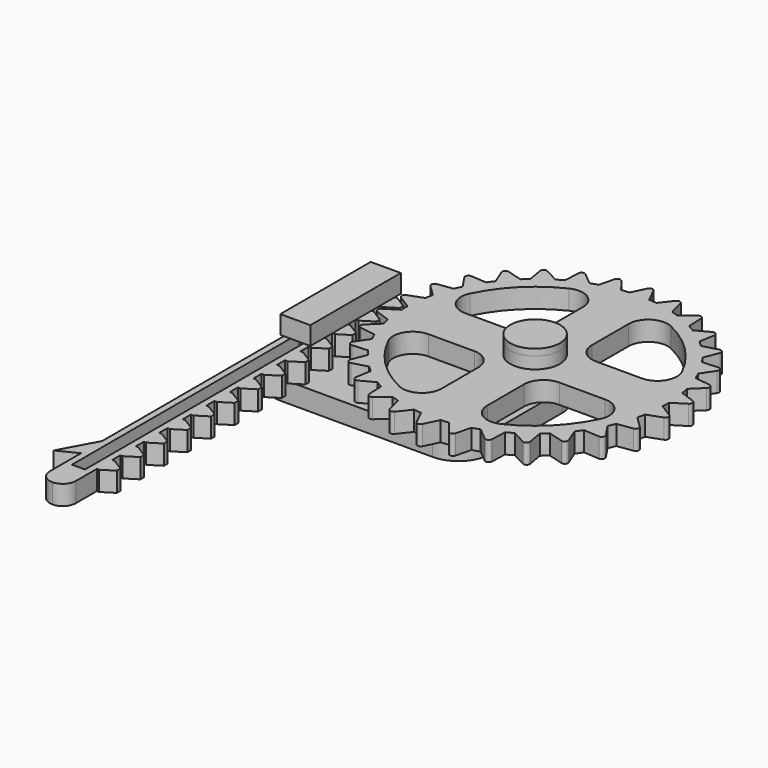
from build123d import *

# Parameters (mm, degrees)
F1_DEPTH        = 3
F2_DEPTH        = 3
F2_COPIES_COUNT = 30
F3_R            = 0.5
F5_DEPTH        = 3
F6_W            = 2
F6_H            = 57.4811261014
F7_DEPTH        = 3.001
F8_T1_DEPTH     = 12.7063351407
F8_T3_DEPTH     = 13
F9_R            = 18
F10_DEPTH       = 3.001
F11_W           = 15
F11_H           = 7
F11_W_2         = 7
F11_H_2         = 15
F12_DEPTH       = 3
F13_R           = 2.5
F14_DEPTH       = 3.001
F15_R           = 3
F16_W           = 33.1953612559
F16_H           = 23.5
F17_DEPTH       = 3
F18_W           = 1.3
F18_H           = 14
F19_DEPTH       = 5
F20_R           = 5
F21_R           = 2.15
F22_DEPTH       = 5
F23_R           = 3.8
F23_R_2         = 2.3
F24_DEPTH       = 1.8
F25_R           = 3.8
F26_DEPTH       = 1
F27_W           = 4.6
F27_H           = 17.3
F27_W_2         = 1.6
F27_H_2         = 14.3
F28_DEPTH       = 1.8
F29_W           = 4.6
F29_H           = 17.3
F30_DEPTH       = 1
F32_DEPTH       = 3
F34_DEPTH       = 3
F35_W           = 1
F35_H           = 1
F36_DEPTH       = 1


# Not quite as in the source:
# - a fillet or chamfer that OpenCascade refuses, or shapes differently, is made with other operations: its cross-section is extruded or revolved along the edge and cut away or added
# - a pattern or mirror of a feature is missing from the dataset's text; its kind, count and spacing are read off the source's solid


with BuildPart() as f1:
    # F0 (on Top) → F1 (new body)
    with BuildSketch(Plane.XY):
        with BuildLine():
            ThreePointArc((-1.5, 19.9436706752), (-13.6014705087, -14.6628782986), (20, 0))
            ThreePointArc((20, 0), (14.6628782986, 13.6014705087), (1.5, 19.9436706752))
            ThreePointArc((1.5, 19.9436706752), (0, 20), (-1.5, 19.9436706752))
        make_face()
    extrude(amount=F1_DEPTH)

    # F0 (on Top) → F2 (join)
    with BuildSketch(Plane.XY):
        with BuildLine():
            ThreePointArc((-1.5, 19.9436706752), (0, 20), (1.5, 19.9436706752))
            Line((1.5, 19.9436706752), (0, 23))
            Line((0, 23), (-1.5, 19.9436706752))
        make_face()
    f2 = extrude(amount=F2_DEPTH)

    # F2_copies: F2 ×30 about axis
    f2_copies_axis = Axis((0, 0, 0), (0, 0, 1))
    for i in range(1, F2_COPIES_COUNT):
        add(f2.rotate(f2_copies_axis, i * 360 / F2_COPIES_COUNT))

    # F3
    f3_edges = [f1.edges().sort_by_distance(p)[0] for p in [
        (0, 23, 1.5),
        (22.874004, -2.404155, 1.5),
        (22.874004, 2.404155, 1.5),
        (21.8743, 7.107391, 1.5),
        (19.918584, 11.5, 1.5),
        (17.092331, 15.390004, 1.5),
        (13.519061, 18.607391, 1.5),
        (9.354943, 21.011546, 1.5),
        (-4.781969, 22.497395, 1.5),
        (-9.354943, 21.011546, 1.5),
        (-13.519061, 18.607391, 1.5),
        (-17.092331, 15.390004, 1.5),
        (-19.918584, 11.5, 1.5),
        (-21.8743, 7.107391, 1.5),
        (-22.874004, 2.404155, 1.5),
        (-22.874004, -2.404155, 1.5),
        (-21.8743, -7.107391, 1.5),
        (-19.918584, -11.5, 1.5),
        (-17.092331, -15.390004, 1.5),
        (-13.519061, -18.607391, 1.5),
        (-9.354943, -21.011546, 1.5),
        (-4.781969, -22.497395, 1.5),
        (0, -23, 1.5),
        (4.781969, -22.497395, 1.5),
        (9.354943, -21.011546, 1.5),
        (13.519061, -18.607391, 1.5),
        (17.092331, -15.390004, 1.5),
        (19.918584, -11.5, 1.5),
        (21.8743, -7.107391, 1.5),
        (4.781969, 22.497395, 1.5),
    ]]
    fillet(f3_edges, radius=F3_R)

    # F9 (on face) → F10 (cut, through all)
    with BuildSketch(Plane.XY.offset(3)):
        Circle(F9_R)
    extrude(amount=-F10_DEPTH, mode=Mode.SUBTRACT)

    # F11 (on Top) → F12 (join)
    with BuildSketch(Plane.XY):
        with Locations((-11, 0)):
            Rectangle(F11_W, F11_H)
        with Locations((0, 11)):
            Rectangle(F11_W_2, F11_H_2)
        Rectangle(F11_W_2, F11_H)
        with Locations((0, -11)):
            Rectangle(F11_W_2, F11_H_2)
        with Locations((11, 0)):
            Rectangle(F11_W, F11_H)
    extrude(amount=F12_DEPTH)

    # F13 (on face) → F14 (cut, through all)
    with BuildSketch(Plane.XY.offset(3)):
        Circle(F13_R)
    extrude(amount=-F14_DEPTH, mode=Mode.SUBTRACT)

    # F15
    f15_edges = [f1.edges().sort_by_distance(p)[0] for p in [
        (3.5, 17.656444, 1.5),
        (3.5, -3.5, 1.5),
        (-3.5, -3.5, 1.5),
        (17.656444, -3.5, 1.5),
        (3.5, -17.656444, 1.5),
        (-17.656444, -3.5, 1.5),
        (-3.5, -17.656444, 1.5),
        (-3.5, 3.5, 1.5),
        (3.5, 3.5, 1.5),
        (-17.656444, 3.5, 1.5),
        (-3.5, 17.656444, 1.5),
        (17.656444, 3.5, 1.5),
    ]]
    fillet(f15_edges, radius=F15_R)


with BuildPart() as f5:
    # F4 (on Top) → F5 (new body)
    with BuildSketch(Plane.XY):
        Polygon((-26.6953612559, 3), (-26.6953612559, -61.4811261014), (-22.6953612559, -61.4811261014), (-22.6953612559, -55.4810394768), (-22.6953612559, -52.518787274), (-22.6953612559, -50.9810466955), (-22.6953612559, -48.0187944927), (-22.6953612559, -46.4810539142), (-22.6953612559, -43.5188017114), (-22.6953612559, -41.9810611329), (-22.6953612559, -39.0188089301), (-22.6953612559, -37.4810683516), (-22.6953612559, -34.5188161489), (-22.6953612559, -32.9810755704), (-22.6953612559, -30.0188233676), (-22.6953612559, -28.4810827891), (-22.6953612559, -25.5188305863), (-22.6953612559, -23.9810900078), (-22.6953612559, -21.018837805), (-22.6953612559, -19.4810972265), (-22.6953612559, -16.5188450237), (-22.6953612559, -14.9811044452), (-22.6953612559, -12.0188522425), (-22.6953612559, -10.4811116639), (-22.6953612559, -7.5188594612), (-22.6953612559, -5.9811188827), (-22.6953612559, -3.0188666799), (-22.6953612559, -1.4811261014), (-22.6953612559, 1.4811261014), (-22.6953612559, 3), align=None)
        with BuildLine():
            Line((-22.6953612559, -52.518787274), (-22.6953612559, -55.4810394768))
            Line((-22.6953612559, -55.4810394768), (-22.3474906883, -55.4810394768))
            Line((-22.3474906883, -55.4810394768), (-20.5437649967, -54.3477605362))
            ThreePointArc((-20.5437649967, -54.3477605362), (-20.5467235884, -53.9999133754), (-20.5437649967, -53.6520662145))
            Line((-20.5437649967, -53.6520662145), (-22.3474906883, -52.518787274))
            Line((-22.3474906883, -52.518787274), (-22.6953612559, -52.518787274))
        make_face()
        with BuildLine():
            Line((-22.2507670999, 1.4811261014), (-22.6953612559, 1.4811261014))
            Line((-22.6953612559, 1.4811261014), (-22.6953612559, -1.4811261014))
            Line((-22.6953612559, -1.4811261014), (-22.2507670999, -1.4811261014))
            Line((-22.2507670999, -1.4811261014), (-20.4470414083, -0.3478471608))
            ThreePointArc((-20.4470414083, -0.3478471608), (-20.45, 0), (-20.4470414083, 0.3478471608))
            Line((-20.4470414083, 0.3478471608), (-22.2507670999, 1.4811261014))
        make_face()
        with BuildLine():
            Line((-22.6953612559, -48.0187944927), (-22.6953612559, -50.9810466955))
            Line((-22.6953612559, -50.9810466955), (-22.3394303893, -50.9810466955))
            Line((-22.3394303893, -50.9810466955), (-20.5357046977, -49.8477677549))
            ThreePointArc((-20.5357046977, -49.8477677549), (-20.5386632894, -49.4999205941), (-20.5357046977, -49.1520734333))
            Line((-20.5357046977, -49.1520734333), (-22.3394303893, -48.0187944927))
            Line((-22.3394303893, -48.0187944927), (-22.6953612559, -48.0187944927))
        make_face()
        with BuildLine():
            Line((-22.2588273989, -3.0188666799), (-22.6953612559, -3.0188666799))
            Line((-22.6953612559, -3.0188666799), (-22.6953612559, -5.9811188827))
            Line((-22.6953612559, -5.9811188827), (-22.2588273989, -5.9811188827))
            Line((-22.2588273989, -5.9811188827), (-20.4551017073, -4.8478399421))
            ThreePointArc((-20.4551017073, -4.8478399421), (-20.458060299, -4.4999927813), (-20.4551017073, -4.1521456204))
            Line((-20.4551017073, -4.1521456204), (-22.2588273989, -3.0188666799))
        make_face()
        with BuildLine():
            Line((-22.6953612559, -43.5188017114), (-22.6953612559, -46.4810539142))
            Line((-22.6953612559, -46.4810539142), (-22.3313700903, -46.4810539142))
            Line((-22.3313700903, -46.4810539142), (-20.5276443986, -45.3477749736))
            ThreePointArc((-20.5276443986, -45.3477749736), (-20.5306029903, -44.9999278128), (-20.5276443986, -44.652080652))
            Line((-20.5276443986, -44.652080652), (-22.3313700903, -43.5188017114))
            Line((-22.3313700903, -43.5188017114), (-22.6953612559, -43.5188017114))
        make_face()
        with BuildLine():
            Line((-22.266887698, -7.5188594612), (-22.6953612559, -7.5188594612))
            Line((-22.6953612559, -7.5188594612), (-22.6953612559, -10.4811116639))
            Line((-22.6953612559, -10.4811116639), (-22.266887698, -10.4811116639))
            Line((-22.266887698, -10.4811116639), (-20.4631620064, -9.3478327234))
            ThreePointArc((-20.4631620064, -9.3478327234), (-20.4661205981, -8.9999855626), (-20.4631620064, -8.6521384017))
            Line((-20.4631620064, -8.6521384017), (-22.266887698, -7.5188594612))
        make_face()
        with BuildLine():
            Line((-22.6953612559, -39.0188089301), (-22.6953612559, -41.9810611329))
            Line((-22.6953612559, -41.9810611329), (-22.3233097912, -41.9810611329))
            Line((-22.3233097912, -41.9810611329), (-20.5195840996, -40.8477821924))
            ThreePointArc((-20.5195840996, -40.8477821924), (-20.5225426913, -40.4999350315), (-20.5195840996, -40.1520878707))
            Line((-20.5195840996, -40.1520878707), (-22.3233097912, -39.0188089301))
            Line((-22.3233097912, -39.0188089301), (-22.6953612559, -39.0188089301))
        make_face()
        with BuildLine():
            Line((-22.274947997, -12.0188522425), (-22.6953612559, -12.0188522425))
            Line((-22.6953612559, -12.0188522425), (-22.6953612559, -14.9811044452))
            Line((-22.6953612559, -14.9811044452), (-22.274947997, -14.9811044452))
            Line((-22.274947997, -14.9811044452), (-20.4712223054, -13.8478255047))
            ThreePointArc((-20.4712223054, -13.8478255047), (-20.4741808971, -13.4999783438), (-20.4712223054, -13.152131183))
            Line((-20.4712223054, -13.152131183), (-22.274947997, -12.0188522425))
        make_face()
        with BuildLine():
            Line((-22.6953612559, -34.5188161489), (-22.6953612559, -37.4810683516))
            Line((-22.6953612559, -37.4810683516), (-22.3152494922, -37.4810683516))
            Line((-22.3152494922, -37.4810683516), (-20.5115238006, -36.3477894111))
            ThreePointArc((-20.5115238006, -36.3477894111), (-20.5144823923, -35.9999422502), (-20.5115238006, -35.6520950894))
            Line((-20.5115238006, -35.6520950894), (-22.3152494922, -34.5188161489))
            Line((-22.3152494922, -34.5188161489), (-22.6953612559, -34.5188161489))
        make_face()
        with BuildLine():
            Line((-22.2830082961, -16.5188450237), (-22.6953612559, -16.5188450237))
            Line((-22.6953612559, -16.5188450237), (-22.6953612559, -19.4810972265))
            Line((-22.6953612559, -19.4810972265), (-22.2830082961, -19.4810972265))
            Line((-22.2830082961, -19.4810972265), (-20.4792826044, -18.347818286))
            ThreePointArc((-20.4792826044, -18.347818286), (-20.4822411961, -17.9999711251), (-20.4792826044, -17.6521239643))
            Line((-20.4792826044, -17.6521239643), (-22.2830082961, -16.5188450237))
        make_face()
        with BuildLine():
            Line((-22.6953612559, -30.0188233676), (-22.6953612559, -32.9810755704))
            Line((-22.6953612559, -32.9810755704), (-22.3071891932, -32.9810755704))
            Line((-22.3071891932, -32.9810755704), (-20.5034635015, -31.8477966298))
            ThreePointArc((-20.5034635015, -31.8477966298), (-20.5064220932, -31.499949469), (-20.5034635015, -31.1521023081))
            Line((-20.5034635015, -31.1521023081), (-22.3071891932, -30.0188233676))
            Line((-22.3071891932, -30.0188233676), (-22.6953612559, -30.0188233676))
        make_face()
        with BuildLine():
            Line((-22.2910685951, -21.018837805), (-22.6953612559, -21.018837805))
            Line((-22.6953612559, -21.018837805), (-22.6953612559, -23.9810900078))
            Line((-22.6953612559, -23.9810900078), (-22.2910685951, -23.9810900078))
            Line((-22.2910685951, -23.9810900078), (-20.4873429035, -22.8478110672))
            ThreePointArc((-20.4873429035, -22.8478110672), (-20.4903014952, -22.4999639064), (-20.4873429035, -22.1521167456))
            Line((-20.4873429035, -22.1521167456), (-22.2910685951, -21.018837805))
        make_face()
        with BuildLine():
            Line((-22.6953612559, -25.5188305863), (-22.6953612559, -28.4810827891))
            Line((-22.6953612559, -28.4810827891), (-22.2991288941, -28.4810827891))
            Line((-22.2991288941, -28.4810827891), (-20.4954032025, -27.3478038485))
            ThreePointArc((-20.4954032025, -27.3478038485), (-20.4983617942, -26.9999566877), (-20.4954032025, -26.6521095268))
            Line((-20.4954032025, -26.6521095268), (-22.2991288941, -25.5188305863))
            Line((-22.2991288941, -25.5188305863), (-22.6953612559, -25.5188305863))
        make_face()
    extrude(amount=F5_DEPTH)

    # F6 (on face) → F7 (cut, through all)
    with BuildSketch(Plane(origin=(0, 0, 0), x_dir=(1, 0, 0), z_dir=(0, 0, -1))):
        with Locations((-24.6953612559, 27.7405630507)):
            Rectangle(F6_W, F6_H)
    extrude(amount=-F7_DEPTH, mode=Mode.SUBTRACT)

    # F8: fillet of radius 2 on 4 edges, made by hand

    # F8_s2 → F8_t1 (cut)
    with BuildSketch(Plane.XY.offset(-4.8531675704)):
        with BuildLine():
            ThreePointArc((-24.6366282841, 3), (-23.4042022625, 2.5751590718), (-22.6953612559, 1.4811261014))
            Line((-22.6953612559, 1.4811261014), (-22.6953612559, 3))
            Line((-22.6953612559, 3), (-24.6366282841, 3))
        make_face()
    extrude(amount=F8_T1_DEPTH, mode=Mode.SUBTRACT)

    # F8_s4 → F8_t3 (cut)
    with BuildSketch(Plane.XY.offset(-5)):
        with BuildLine():
            ThreePointArc((-24.6953612559, 3), (-26.1095748183, 2.4142135624), (-26.6953612559, 1))
            Line((-26.6953612559, 1), (-26.6953612559, 3))
            Line((-26.6953612559, 3), (-24.6953612559, 3))
        make_face()
        with BuildLine():
            ThreePointArc((-26.6953612559, -59.4811261014), (-26.1095748183, -60.8953396638), (-24.6953612559, -61.4811261014))
            Line((-24.6953612559, -61.4811261014), (-26.6953612559, -61.4811261014))
            Line((-26.6953612559, -61.4811261014), (-26.6953612559, -59.4811261014))
        make_face()
        with BuildLine():
            ThreePointArc((-24.6953612559, -61.4811261014), (-23.2811476936, -60.8953396638), (-22.6953612559, -59.4811261014))
            Line((-22.6953612559, -59.4811261014), (-22.6953612559, -61.4811261014))
            Line((-22.6953612559, -61.4811261014), (-24.6953612559, -61.4811261014))
        make_face()
    extrude(amount=F8_T3_DEPTH, mode=Mode.SUBTRACT)

    # F31 (on Top) → F32 (join)
    with BuildSketch(Plane.XY):
        Polygon((-26.6953612559, -53.4811261014), (-26.6953612559, -49.4427494705), (-29.6953612559, -54.9811261014), align=None)
    extrude(amount=F32_DEPTH)


with BuildPart() as f17:
    # F16 (on Top) → F17 (new body)
    with BuildSketch(Plane.XY):
        with Locations((-12.097680628, -7.25)):
            Rectangle(F16_W, F16_H)
    extrude(amount=-F17_DEPTH)

    # F18 (on face) → F19 (join)
    with BuildSketch(Plane.XY):
        with Locations((-24.6953612559, -6.35)):
            Rectangle(F18_W, F18_H)
    extrude(amount=F19_DEPTH)

    # F20
    f20_edges = [f17.edges().sort_by_distance(p)[0] for p in [
        (4.5, -19, -1.5),
        (4.5, 4.5, -1.5),
        (-28.695361, 4.5, -1.5),
        (-28.695361, -19, -1.5),
    ]]
    fillet(f20_edges, radius=F20_R)

    # F21 (on face) → F22 (join)
    with BuildSketch(Plane.XY):
        Circle(F21_R)
    extrude(amount=F22_DEPTH)

    # F33 (on Top) → F34 (join)
    with BuildSketch(Plane.XY):
        Polygon((-30.6953612559, -2), (-30.6953612559, -0.5), (-32.1953612559, -0.5), (-32.1953612559, -3.5), (-28.6953612559, -3.5), (-28.6953612559, -2), align=None)
    extrude(amount=-F34_DEPTH)

    # F35 (on face) → F36 (join)
    with BuildSketch(Plane.XY):
        with Locations((-27.5953612559, -13.5)):
            Rectangle(F35_W, F35_H)
    extrude(amount=F36_DEPTH)


with BuildPart() as f24:
    # F23 (on face) → F24 (new body)
    with BuildSketch(Plane.XY.offset(5)):
        Circle(F23_R)
        Circle(F23_R_2, mode=Mode.SUBTRACT)
    extrude(amount=-F24_DEPTH)

    # F25 (on face) → F26 (join)
    with BuildSketch(Plane.XY.offset(5)):
        Circle(F25_R)
    extrude(amount=F26_DEPTH)


with BuildPart() as f28:
    # F27 (on face) → F28 (new body)
    with BuildSketch(Plane.XY.offset(5)):
        with Locations((-24.6953612559, -6.35)):
            Rectangle(F27_W, F27_H)
        with Locations((-24.6953612559, -6.35)):
            Rectangle(F27_W_2, F27_H_2, mode=Mode.SUBTRACT)
    extrude(amount=-F28_DEPTH)

    # F29 (on face) → F30 (join)
    with BuildSketch(Plane.XY.offset(5)):
        with Locations((-24.6953612559, -6.35)):
            Rectangle(F29_W, F29_H)
    extrude(amount=F30_DEPTH)


solid = Compound([f1.part, f5.part, f17.part, f24.part, f28.part])
